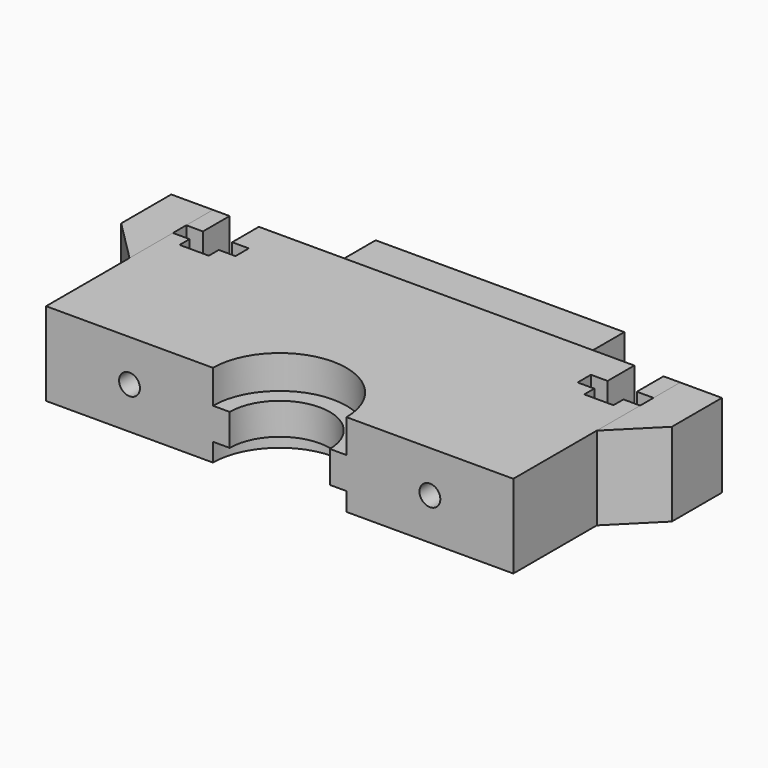
from build123d import *

# Parameters (mm, degrees)
F0_W       = 56
F0_H       = 25
F1_DEPTH   = 10
F3_DEPTH   = 25
F5_DEPTH   = 25
F6_R       = 6
F7_DEPTH   = 25
F8_R       = 8
F9_DEPTH   = 4
F10_R      = 8
F11_DEPTH  = 2.2
F13_D      = 2.5
F13_DEPTH  = 12
F13_TIP    = 0.7510757738
F14_W      = 15
F14_H      = 5
F15_DEPTH  = 5
F16_SIZE   = 4.99999
F17_W      = 5
F17_H      = 12.5
F18_DEPTH  = 10
F19_SIZE   = 4.99999
F19_2_SIZE = 4.99999
F20_W      = 29.8
F20_H      = 7.8
F21_DEPTH  = 8


# Not quite as in the source:
# - a fillet or chamfer is up to 0.001 mm smaller than in the source, because OpenCascade refuses the exact size


with BuildPart() as f1:
    # F0 (on Top) → F1 (new body)
    with BuildSketch(Plane.XY):
        with Locations((2.6210285723, -1.1366620937)):
            Rectangle(F0_W, F0_H)
    extrude(amount=F1_DEPTH)

    # F2 (on face) → F3 (cut)
    with BuildSketch(Plane.XY.offset(10)):
        Polygon((28.6210285723, 7.3633379063), (28.6210285723, 11.3633379063), (25.1210285723, 11.3633379063), (25.1210285723, 7.3633379063), (23.1210285723, 7.3633379063), (23.1210285723, 5.3633379063), (25.1210285723, 5.3633379063), (25.1210285723, 3.8633379063), (28.6210285723, 3.8633379063), (28.6210285723, 5.3633379063), (30.6210285723, 5.3633379063), (30.6210285723, 7.3633379063), align=None)
    extrude(amount=-F3_DEPTH, mode=Mode.SUBTRACT)

    # F4 (on face) → F5 (cut)
    with BuildSketch(Plane.XY.offset(10)):
        Polygon((-19.8789714277, 7.3633379063), (-19.8789714277, 11.3633379063), (-23.3789714277, 11.3633379063), (-23.3789714277, 7.3633379063), (-25.3789714277, 7.3633379063), (-25.3789714277, 5.3633379063), (-23.3789714277, 5.3633379063), (-23.3789714277, 3.8633379063), (-19.8789714277, 3.8633379063), (-19.8789714277, 5.3633379063), (-17.8789714277, 5.3633379063), (-17.8789714277, 7.3633379063), align=None)
    extrude(amount=-F5_DEPTH, mode=Mode.SUBTRACT)

    # F6 (on face) → F7 (cut)
    with BuildSketch(Plane.XY.offset(10)):
        with Locations((2.6210285723, -13.6366620937)):
            Circle(F6_R)
    extrude(amount=-F7_DEPTH, mode=Mode.SUBTRACT)

    # F8 (on face) → F9 (cut)
    with BuildSketch(Plane.XY.offset(10)):
        with Locations((2.6210285723, -13.6366620937)):
            Circle(F8_R)
    extrude(amount=-F9_DEPTH, mode=Mode.SUBTRACT)

    # F10 (on face) → F11 (cut)
    with BuildSketch(Plane(origin=(0, 0, 0), x_dir=(1, 0, 0), z_dir=(0, 0, -1))):
        with Locations((2.6210285723, 13.6366620937)):
            Circle(F10_R)
    extrude(amount=-F11_DEPTH, mode=Mode.SUBTRACT)

    # F13
    with Locations(Plane.XZ.offset(13.6366620937)):
        with Locations((-15.3789714277, 5), (20.6210285723, 5)):
            Hole(F13_D / 2, depth=F13_DEPTH)
            with Locations((0, 0, -(F13_DEPTH + F13_TIP / 2))):  # 118° drill point
                Cone(0, F13_D / 2, F13_TIP, mode=Mode.SUBTRACT)

    # F14 (on face) → F15 (join)
    with BuildSketch(Plane(origin=(0, 0, 0), x_dir=(1, 0, 0), z_dir=(0, 0, -1))):
        with Locations((2.6210285723, -8.8633379063)):
            Rectangle(F14_W, F14_H)
    extrude(amount=F15_DEPTH)

    # F16 (size 5 in the source; OpenCascade refuses exactly that, so slightly less here)
    f16_edges = [f1.edges().sort_by_distance(p)[0] for p in [
        (2.621029, 6.363338, -5),
    ]]
    chamfer(f16_edges, length=F16_SIZE)

    # F20 (on face) → F21 (join)
    with BuildSketch(Plane(origin=(0, 11.3633379063, 0), x_dir=(-1, 0, 0), z_dir=(0, 1, 0))):
        with Locations((-2.6210285723, 3.9)):
            Rectangle(F20_W, F20_H)
    extrude(amount=F21_DEPTH)


with BuildPart() as f18:
    # F17 (on face) → F18 (new body)
    with BuildSketch(Plane.XY.offset(10)):
        with Locations((-27.8789714277, 5.1133379063)):
            Rectangle(F17_W, F17_H)
    extrude(amount=-F18_DEPTH)

    # F19#2 (size 5 in the source; OpenCascade refuses exactly that, so slightly less here)
    f19_2_edges = [f18.edges().sort_by_distance(p)[0] for p in [
        (-30.378971, -1.136662, 5),
    ]]
    chamfer(f19_2_edges, length=F19_2_SIZE)


with BuildPart() as f18b:
    # F17 (on face) → F18, piece 2 (new body)
    with BuildSketch(Plane.XY.offset(10)):
        with Locations((33.1210285723, 5.1133379063)):
            Rectangle(F17_W, F17_H)
    extrude(amount=-F18_DEPTH)

    # F19 (size 5 in the source; OpenCascade refuses exactly that, so slightly less here)
    f19_edges = [f18b.edges().sort_by_distance(p)[0] for p in [
        (35.621029, -1.136662, 5),
    ]]
    chamfer(f19_edges, length=F19_SIZE)


solid = Compound([f1.part, f18.part, f18b.part])
